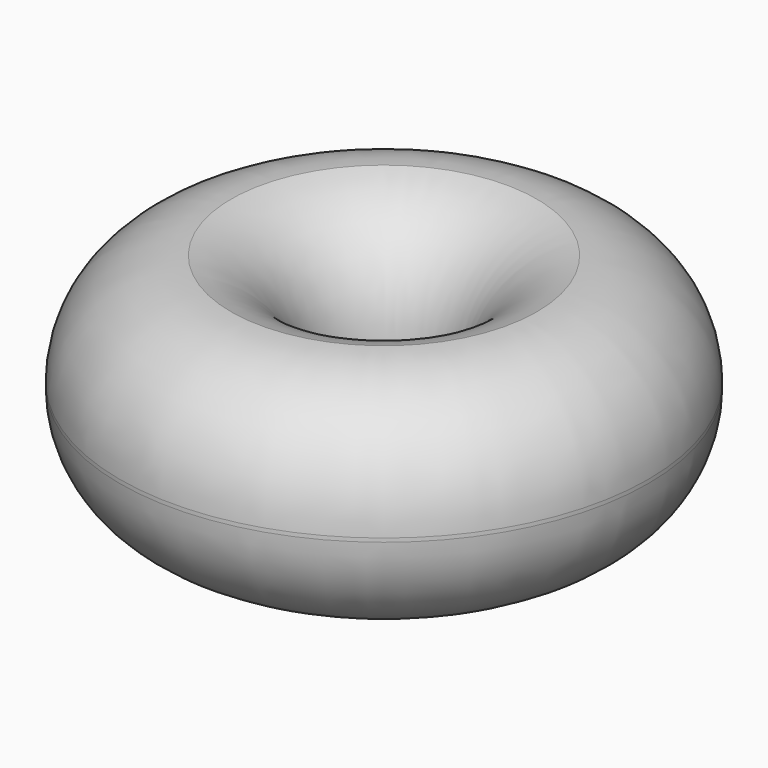
from build123d import *

# Parameters (mm, degrees)
F0_R     = 72.3406344385
F1_DEPTH = 61.9792044163
F2_R     = 17.7569535603
F3_DEPTH = 66.9353306293
F4_R     = 30.48


# Not quite as in the source:
# - a fillet or chamfer that OpenCascade refuses, or shapes differently, is made with other operations: its cross-section is extruded or revolved along the edge and cut away or added


with BuildPart() as f1:
    # F0 (on Top) → F1 (new body)
    with BuildSketch(Plane.XY):
        Circle(F0_R)
    extrude(amount=F1_DEPTH)

    # F2 (on face) → F3 (cut)
    with BuildSketch(Plane.XY.offset(61.9792044163)):
        Circle(F2_R)
    extrude(amount=-F3_DEPTH, mode=Mode.SUBTRACT)

    # F4
    f4_edges = [f1.edges().sort_by_distance(p)[0] for p in [
        (-72.340634, 0, 61.979204),
        (72.340634, 0, 30.989602),
        (-72.340634, 0, 0),
    ]]
    fillet(f4_edges, radius=F4_R)

    # F5: fillet of radius 30.48 on 3 edges, made by hand

    # F5_s1 → F5_t2 (revolve, cut)
    with BuildSketch(Plane.XZ):
        with BuildLine():
            ThreePointArc((41.8606344385, 61.9792044163), (24.5369471591, 51.3397369094), (17.7569535603, 32.1736184556))
            Line((17.7569535603, 32.1736184556), (17.7569535603, 61.9792044163))
            Line((17.7569535603, 61.9792044163), (41.8606344385, 61.9792044163))
        make_face()
    revolve(axis=Axis((0, 0, 61.9792044163), (0, 0, 1)), mode=Mode.SUBTRACT)

    # F5_s3 → F5_t4 (revolve, cut)
    with BuildSketch(Plane.XZ):
        with BuildLine():
            ThreePointArc((41.8606344385, 0), (24.5369471591, 10.6394675069), (17.7569535603, 29.8055859606))
            Line((17.7569535603, 29.8055859606), (17.7569535603, 0))
            Line((17.7569535603, 0), (41.8606344385, 0))
        make_face()
    revolve(axis=Axis((0, 0, 0), (0, 0, 1)), mode=Mode.SUBTRACT)


solid = f1.part
